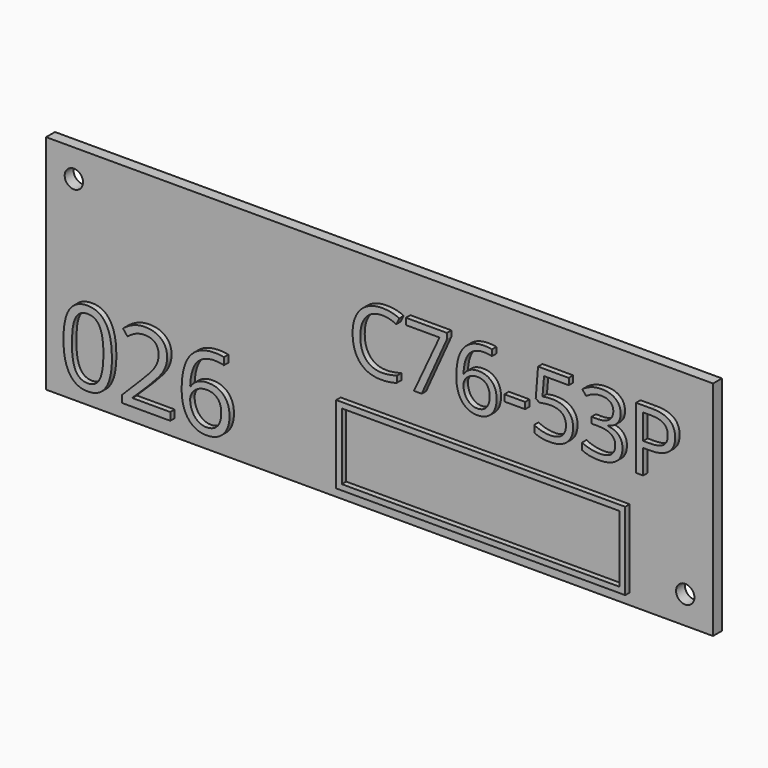
from build123d import *

# Parameters (mm, degrees)
F0_W         = 120
F0_H         = 40
F1_DEPTH     = 2
F3_D         = 3.3
F4_TEXT_SIZE = 15.5635715154
F5_DEPTH     = 1
F6_TEXT_SIZE = 18.4837545126
F7_DEPTH     = 1
F8_W         = 52
F8_H         = 14
F8_W_2       = 49.99999962
F8_H_2       = 11.99999962
F9_DEPTH     = 1


# Not quite as in the source:
# - Text() gives the source's letters only with a copy of the font that has no kerning and outlines rounded to 1/6400 em; it was checked with that copy


with BuildPart() as f1:
    # F0 (on Front) → F1 (new body)
    with BuildSketch(Plane.XZ):
        Rectangle(F0_W, F0_H)
    extrude(amount=F1_DEPTH)

    # F3 (through all)
    with Locations(Plane.XZ.offset(2)):
        with Locations((-55, 15), (55, -15)):
            Hole(F3_D / 2)

    # F4 (on face) → F5 (join)
    with BuildSketch(Plane.XZ.offset(2)):
        with Locations((-5, 2)):
            Text('C76-53P', F4_TEXT_SIZE, font='Open Sans', text_align=(TextAlign.LEFT, TextAlign.BOTTOM))
    extrude(amount=F5_DEPTH)

    # F6 (on face) → F7 (join)
    with BuildSketch(Plane.XZ.offset(2)):
        with Locations((-57, -17)):
            Text('026', F6_TEXT_SIZE, font='Open Sans', text_align=(TextAlign.LEFT, TextAlign.BOTTOM))
    extrude(amount=F7_DEPTH)

    # F8 (on face) → F9 (join)
    with BuildSketch(Plane.XZ.offset(2)):
        with Locations((19, -11)):
            Rectangle(F8_W, F8_H)
        with Locations((19, -11)):
            Rectangle(F8_W_2, F8_H_2, mode=Mode.SUBTRACT)
    extrude(amount=F9_DEPTH)


solid = f1.part
